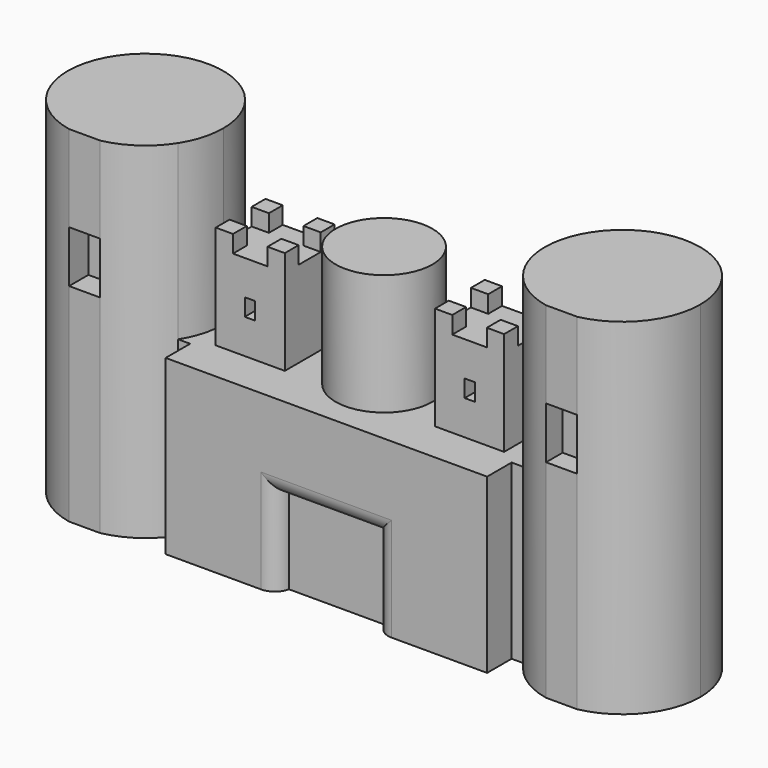
from build123d import *

# Parameters (mm, degrees)
F1_DEPTH     = 100
F0_R         = 14
F2_DEPTH     = 50
F3_DEPTH     = 75
F4_DEPTH     = 85
F0_W         = 5
F0_H         = 5
F5_DEPTH     = 80
F6_START     = 25
F0_W_2       = 28
F0_H_2       = 3.9854568298
F6_DEPTH     = 25
F7_START     = 75
F0_W_3       = 9
F0_H_3       = 7
F0_H_4       = 6
F7_DEPTH     = 25
F8_DEPTH     = 60
F9_T1_DEPTH  = 28
F9_T3_DEPTH  = 37.2399709343
F9_T9_DEPTH  = 40.2399709343
F9_T13_DEPTH = 37.2399709343
F9_T20_DEPTH = 37.2399709343
F9_T24_DEPTH = 40.2399709343
F10_START    = 65
F0_W_4       = 3
F10_DEPTH    = 10
F11_DEPTH    = 60


# Not quite as in the source:
# - a fillet or chamfer that OpenCascade refuses, or shapes differently, is made with other operations: its cross-section is extruded or revolved along the edge and cut away or added
# - a feature names something its author has since deleted; it is built from what else it names


with BuildPart() as f1:
    # F0 (on Top) → F1 (new body)
    with BuildSketch(Plane.XY):
        with BuildLine():
            ThreePointArc((-49.982315052, -12), (-47.3993365724, -6.2454186413), (-46.5151813626, 0))
            ThreePointArc((-46.5151813626, 0), (-47.3993365724, 6.2454186413), (-49.982315052, 12))
            ThreePointArc((-49.982315052, 12), (-87.5239224573, 12.7936118078), (-73.5151813626, -22.045407685))
            Line((-73.5151813626, -22.045407685), (-73.5151813626, -15.045407685))
            Line((-73.5151813626, -15.045407685), (-64.5151813626, -15.045407685))
            Line((-64.5151813626, -15.045407685), (-64.5151813626, -22.045407685))
            ThreePointArc((-64.5151813626, -22.045407685), (-56.2215695548, -18.5087410947), (-49.982315052, -12))
        make_face()
    extrude(amount=F1_DEPTH)



with BuildPart() as f1b:
    # F0 (on Top) → F1, piece 2 (new body)
    with BuildSketch(Plane.XY):
        with BuildLine():
            ThreePointArc((49.982315052, 12), (47.3993365677, 6.2454186249), (46.5151813626, -3.41e-08))
            ThreePointArc((46.5151813626, -3.41e-08), (47.3993365771, -6.2454186577), (49.982315052, -12))
            ThreePointArc((49.982315052, -12), (56.2215695548, -18.5087410947), (64.5151813626, -22.045407685))
            Line((64.5151813626, -22.045407685), (64.5151813626, -16.045407685))
            Line((64.5151813626, -16.045407685), (73.5151813626, -16.045407685))
            Line((73.5151813626, -16.045407685), (73.5151813626, -22.045407685))
            ThreePointArc((73.5151813626, -22.045407685), (86.4436064206, -14.2302494708), (91.5151813626, 0))
            ThreePointArc((91.5151813626, 0), (75.2606000039, 21.6158447902), (49.982315052, 12))
        make_face()
    extrude(amount=F1_DEPTH)


with BuildPart() as f1_1:
    add(f1.part)

    add(f1b.part)  # F2 merges F1b
    # F0 (on Top) → F2 (join)
    with BuildSketch(Plane.XY):
        Polygon((46.5151813626, 12), (46.5151813626, 20.8604575003), (-46.5151813626, 20.8604575003), (-46.5151813626, 12), (-46.5151813626, 0), (-46.5151813626, -12), (-46.5151813626, -20.8604575003), (-14.0001813626, -20.8604575003), (-14.0001813626, -16.8750006706), (13.9998186374, -16.8750006706), (13.9998186374, -20.8604575003), (46.5151813626, -20.8604575003), (46.5151813626, -12), (46.5151813626, -3.41e-08), align=None)
        Polygon((-26.5151813626, 9), (-21.5151813626, 9), (-21.5151813626, 4), (-21.5151813626, -4), (-21.5151813626, -9), (-26.5151813626, -9), (-30.1052076072, -9), (-33.1052076072, -9), (-36.5151813626, -9), (-41.5151813626, -9), (-41.5151813626, -4), (-41.5151813626, 4), (-41.5151813626, 9), (-36.5151813626, 9), align=None, mode=Mode.SUBTRACT)
        Circle(F0_R, mode=Mode.SUBTRACT)
        Polygon((36.9421700871, 9), (41.9421700871, 9), (41.9421700871, 4), (41.9421700871, -4), (41.9421700871, -9), (36.9421700871, -9), (33.5321700871, -9), (30.5321700871, -9), (26.9421700871, -9), (21.9421700871, -9), (21.9421700871, -4), (21.9421700871, 4), (21.9421700871, 9), (26.9421700871, 9), align=None, mode=Mode.SUBTRACT)
        with BuildLine():
            Line((-46.5151813626, -12), (-46.5151813626, 0))
            ThreePointArc((-46.5151813626, 0), (-47.3993365724, -6.2454186413), (-49.982315052, -12))
            Line((-49.982315052, -12), (-46.5151813626, -12))
        make_face()
        with BuildLine():
            Line((-46.5151813626, 0), (-46.5151813626, 12))
            Line((-46.5151813626, 12), (-49.982315052, 12))
            ThreePointArc((-49.982315052, 12), (-47.3993365724, 6.2454186413), (-46.5151813626, 0))
        make_face()
        with BuildLine():
            ThreePointArc((49.982315052, -12), (47.3993365771, -6.2454186577), (46.5151813626, -3.41e-08))
            Line((46.5151813626, -3.41e-08), (46.5151813626, -12))
            Line((46.5151813626, -12), (49.982315052, -12))
        make_face()
        with BuildLine():
            Line((49.982315052, 12), (46.5151813626, 12))
            Line((46.5151813626, 12), (46.5151813626, -3.41e-08))
            ThreePointArc((46.5151813626, -3.41e-08), (47.3993365677, 6.2454186249), (49.982315052, 12))
        make_face()
    extrude(amount=F2_DEPTH)

    # F0 (on Top) → F3 (join)
    with BuildSketch(Plane.XY):
        Polygon((36.9421700871, 4), (36.9421700871, 9), (26.9421700871, 9), (26.9421700871, 4), (21.9421700871, 4), (21.9421700871, -4), (26.9421700871, -4), (26.9421700871, -9), (30.5321700871, -9), (30.5321700871, -4), (33.5321700871, -4), (33.5321700871, -9), (36.9421700871, -9), (36.9421700871, -4), (41.9421700871, -4), (41.9421700871, 4), align=None)
        Polygon((-26.5151813626, 4), (-26.5151813626, 9), (-36.5151813626, 9), (-36.5151813626, 4), (-41.5151813626, 4), (-41.5151813626, -4), (-36.5151813626, -4), (-36.5151813626, -9), (-33.1052076072, -9), (-33.1052076072, -4), (-30.1052076072, -4), (-30.1052076072, -9), (-26.5151813626, -9), (-26.5151813626, -4), (-21.5151813626, -4), (-21.5151813626, 4), align=None)
    extrude(amount=F3_DEPTH)

    # F0 (on Top) → F4 (join)
    with BuildSketch(Plane.XY):
        Circle(F0_R)
    extrude(amount=F4_DEPTH)

    # F0 (on Top) → F5 (join)
    with BuildSketch(Plane.XY):
        with Locations((-39.0151813626, 6.5)):
            Rectangle(F0_W, F0_H)
        with Locations((-39.0151813626, -6.5)):
            Rectangle(F0_W, F0_H)
        with Locations((-24.0151813626, -6.5)):
            Rectangle(F0_W, F0_H)
        with Locations((-24.0151813626, 6.5)):
            Rectangle(F0_W, F0_H)
        with Locations((24.4421700871, -6.5)):
            Rectangle(F0_W, F0_H)
        with Locations((39.4421700871, -6.5)):
            Rectangle(F0_W, F0_H)
        with Locations((39.4421700871, 6.5)):
            Rectangle(F0_W, F0_H)
        with Locations((24.4421700871, 6.5)):
            Rectangle(F0_W, F0_H)
    extrude(amount=F5_DEPTH)

    # F0 (on Top) → F6 (join)
    with BuildSketch(Plane.XY.offset(F6_START)):
        with Locations((-0.0001813626, -18.8677290854)):
            Rectangle(F0_W_2, F0_H_2)
    extrude(amount=F6_DEPTH)

    # F0 (on Top) → F7 (join)
    with BuildSketch(Plane.XY.offset(F7_START)):
        with Locations((-69.0151813626, -18.545407685)):
            Rectangle(F0_W_3, F0_H_3)
        with Locations((69.0151813626, -19.045407685)):
            Rectangle(F0_W_3, F0_H_4)
    extrude(amount=F7_DEPTH)

    # F0 (on Top) → F8 (join)
    with BuildSketch(Plane.XY):
        with Locations((-69.0151813626, -18.545407685)):
            Rectangle(F0_W_3, F0_H_3)
        with Locations((69.0151813626, -19.045407685)):
            Rectangle(F0_W_3, F0_H_4)
    extrude(amount=F8_DEPTH)

    # F9: fillet of radius 5 on 3 edges, made by hand

    # F9_s2 → F9_t1 (cut)
    with BuildSketch(Plane.YZ.offset(-14.0001813626)):
        with BuildLine():
            ThreePointArc((-20.8604575003, 29.8959883737), (-19.7381317937, 26.7394646412), (-16.8750006706, 25))
            Line((-16.8750006706, 25), (-20.8604575003, 25))
            Line((-20.8604575003, 25), (-20.8604575003, 29.8959883737))
        make_face()
    extrude(amount=F9_T1_DEPTH, mode=Mode.SUBTRACT)

    # F9_s4 → F9_t3 (cut)
    with BuildSketch(Plane.XY.offset(-12.2399709343)):
        with BuildLine():
            ThreePointArc((-18.8961697364, -20.8604575003), (-15.7396460038, -19.7381317937), (-14.0001813626, -16.8750006706))
            Line((-14.0001813626, -16.8750006706), (-14.0001813626, -20.8604575003))
            Line((-14.0001813626, -20.8604575003), (-18.8961697364, -20.8604575003))
        make_face()
        with BuildLine():
            ThreePointArc((18.8958070111, -20.8604575003), (15.7392832785, -19.7381317937), (13.9998186374, -16.8750006706))
            Line((13.9998186374, -16.8750006706), (13.9998186374, -20.8604575003))
            Line((13.9998186374, -20.8604575003), (18.8958070111, -20.8604575003))
        make_face()
    extrude(amount=F9_T3_DEPTH, mode=Mode.SUBTRACT)


with BuildPart() as f9_tool7:
    # F9_s8 → F9_t9 (new body)
    with BuildSketch(Plane.YZ.offset(-26.240152297)):
        with BuildLine():
            ThreePointArc((-20.8604575003, 29.8959883737), (-19.7381317937, 26.7394646412), (-16.8750006706, 25))
            Line((-16.8750006706, 25), (-20.8604575003, 25))
            Line((-20.8604575003, 25), (-20.8604575003, 29.8959883737))
        make_face()
    extrude(amount=F9_T9_DEPTH)

    split(bisect_by=Plane.YZ.offset(-14.0001813626), keep=Keep.BOTTOM)


with BuildPart() as f9_tool11:
    # F9_s12 → F9_t13 (new body)
    with BuildSketch(Plane.XY):
        with BuildLine():
            ThreePointArc((-18.8961697364, -20.8604575003), (-15.7396460038, -19.7381317937), (-14.0001813626, -16.8750006706))
            Line((-14.0001813626, -16.8750006706), (-14.0001813626, -20.8604575003))
            Line((-14.0001813626, -20.8604575003), (-18.8961697364, -20.8604575003))
        make_face()
    extrude(amount=F9_T13_DEPTH)

    split(bisect_by=Plane.XY.offset(25), keep=Keep.TOP)


with BuildPart() as f9_tool7_1:
    add(f9_tool7.part)

    # F9_t15: intersect F9_tool11
    add(f9_tool11.part, mode=Mode.INTERSECT)


with BuildPart() as f1_2:
    add(f1_1.part)

    # F9_t5: cut F9_tool7
    add(f9_tool7_1.part, mode=Mode.SUBTRACT)


with BuildPart() as f9_tool18:
    # F9_s19 → F9_t20 (new body)
    with BuildSketch(Plane.XY):
        with BuildLine():
            ThreePointArc((18.8958070111, -20.8604575003), (15.7392832785, -19.7381317937), (13.9998186374, -16.8750006706))
            Line((13.9998186374, -16.8750006706), (13.9998186374, -20.8604575003))
            Line((13.9998186374, -20.8604575003), (18.8958070111, -20.8604575003))
        make_face()
    extrude(amount=F9_T20_DEPTH)

    split(bisect_by=Plane.XY.offset(25), keep=Keep.TOP)


with BuildPart() as f9_tool22:
    # F9_s23 → F9_t24 (new body)
    with BuildSketch(Plane.YZ.offset(-14.0001813626)):
        with BuildLine():
            ThreePointArc((-20.8604575003, 29.8959883737), (-19.7381317937, 26.7394646412), (-16.8750006706, 25))
            Line((-16.8750006706, 25), (-20.8604575003, 25))
            Line((-20.8604575003, 25), (-20.8604575003, 29.8959883737))
        make_face()
    extrude(amount=F9_T24_DEPTH)

    split(bisect_by=Plane.YZ.offset(13.9998186374), keep=Keep.TOP)


with BuildPart() as f9_tool18_1:
    add(f9_tool18.part)

    # F9_t26: intersect F9_tool22
    add(f9_tool22.part, mode=Mode.INTERSECT)


with BuildPart() as f1_3:
    add(f1_2.part)

    # F9_t16: cut F9_tool18
    add(f9_tool18_1.part, mode=Mode.SUBTRACT)

    # F0 (on Top) → F10 (join)
    with BuildSketch(Plane.XY.offset(F10_START)):
        with Locations((-31.6052076072, -6.5)):
            Rectangle(F0_W_4, F0_H)
        with Locations((32.0321700871, -6.5)):
            Rectangle(F0_W_4, F0_H)
    extrude(amount=F10_DEPTH)

    # F0 (on Top) → F11 (join)
    with BuildSketch(Plane.XY):
        with Locations((-31.6052076072, -6.5)):
            Rectangle(F0_W_4, F0_H)
        with Locations((32.0321700871, -6.5)):
            Rectangle(F0_W_4, F0_H)
    extrude(amount=F11_DEPTH)


solid = f1_3.part
